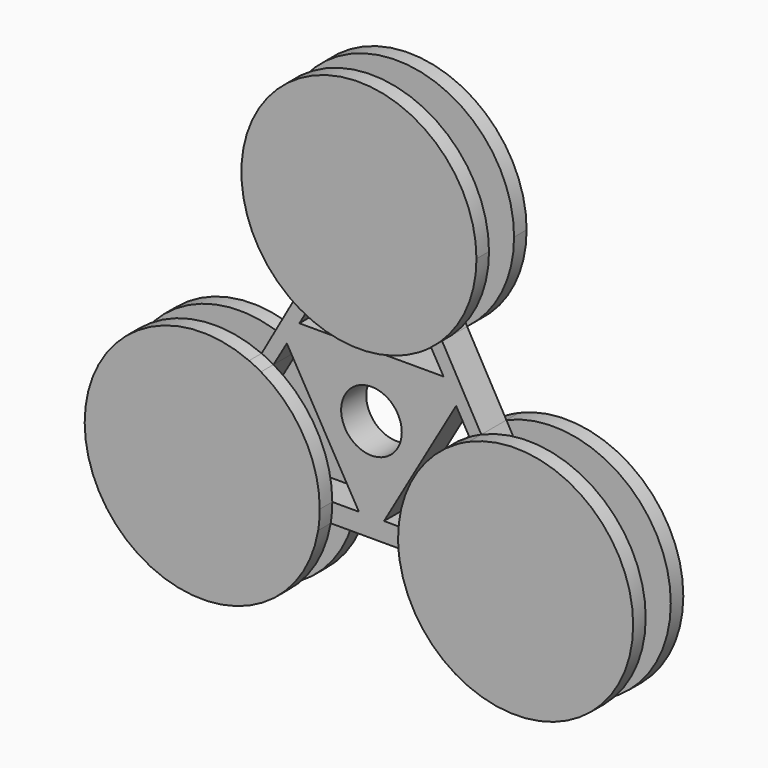
from build123d import *
from build123d import SkipClean  # not in build123d's __all__

# Parameters (mm, degrees)
F0_R     = 4.9113239183
F1_DEPTH = 5.08
F2_DEPTH = 2.54
F4_DEPTH = 2.54
F5_DEPTH = 5.08


# Not quite as in the source:
# - a feature names something its author has since deleted; it is built from what else it names


with BuildPart() as f1:
    # F0 (on Front) → F1 (new body)
    with BuildSketch(Plane.XZ):
        Polygon((11.684, -8.5716721153), (-11.684, -8.5716721153), (-12.7, -10.3314357358), (-13.716, -12.0911993563), (-2.032, -32.3284809919), (0, -32.3284809919), (2.032, -32.3284809919), (13.716, -12.0911993563), (12.7, -10.3314357358), align=None)
        with Locations((0, -18.7316721153)):
            Circle(F0_R, mode=Mode.SUBTRACT)
        with BuildLine():
            ThreePointArc((-11.4414768653, -3.5657760746), (-10.5023439874, -4.227888231), (-9.525, -4.8321744218))
            Line((-9.525, -4.8321744218), (0, 11.6656095203))
            Line((0, 11.6656095203), (0, 16.7456095203))
            Line((0, 16.7456095203), (-11.4414768653, -3.5657760746))
        make_face()
        with BuildLine():
            Line((9.525, -4.8321744218), (11.684, -8.5716721153))
            Line((11.684, -8.5716721153), (12.7, -10.3314357358))
            Line((12.7, -10.3314357358), (13.716, -12.0911993563))
            Line((13.716, -12.0911993563), (15.875, -15.8306970498))
            ThreePointArc((15.875, -15.8306970498), (16.8251832643, -15.3174546282), (17.8029235649, -14.8588808351))
            Line((17.8029235649, -14.8588808351), (11.4414768653, -3.5657760746))
            ThreePointArc((11.4414768653, -3.5657760746), (10.5023439874, -4.227888231), (9.525, -4.8321744218))
        make_face()
        with BuildLine():
            Line((0, 16.7456095203), (0, 11.6656095203))
            Line((0, 11.6656095203), (9.525, -4.8321744218))
            ThreePointArc((9.525, -4.8321744218), (10.5023439874, -4.227888231), (11.4414768653, -3.5657760746))
            Line((11.4414768653, -3.5657760746), (0, 16.7456095203))
        make_face()
        with BuildLine():
            Line((-25.4, -32.3284809919), (-15.875, -15.8306970498))
            ThreePointArc((-15.875, -15.8306970498), (-16.8251832643, -15.3174546282), (-17.8029235649, -14.8588808351))
            Line((-17.8029235649, -14.8588808351), (-29.4044214139, -35.4543423357))
            Line((-29.4044214139, -35.4543423357), (-25.4, -32.3284809919))
        make_face()
        with BuildLine():
            Line((0, -32.3284809919), (-2.032, -32.3284809919))
            Line((-2.032, -32.3284809919), (-6.35, -32.3284809919))
            ThreePointArc((-6.35, -32.3284809919), (-6.4146614456, -33.8967347902), (-6.6082068216, -35.4543423357))
            Line((-6.6082068216, -35.4543423357), (6.6082068216, -35.4543423357))
            ThreePointArc((6.6082068216, -35.4543423357), (6.4146614456, -33.8967347902), (6.35, -32.3284809919))
            Line((6.35, -32.3284809919), (2.032, -32.3284809919))
            Line((2.032, -32.3284809919), (0, -32.3284809919))
        make_face()
        with BuildLine():
            Line((-6.35, -32.3284809919), (-25.4, -32.3284809919))
            Line((-25.4, -32.3284809919), (-29.4044214139, -35.4543423357))
            Line((-29.4044214139, -35.4543423357), (-6.6082068216, -35.4543423357))
            ThreePointArc((-6.6082068216, -35.4543423357), (-6.4146614456, -33.8967347902), (-6.35, -32.3284809919))
        make_face()
        with BuildLine():
            Line((29.4044214139, -35.4543423357), (17.8029235649, -14.8588808351))
            ThreePointArc((17.8029235649, -14.8588808351), (16.8251832643, -15.3174546282), (15.875, -15.8306970498))
            Line((15.875, -15.8306970498), (25.4, -32.3284809919))
            Line((25.4, -32.3284809919), (29.4044214139, -35.4543423357))
        make_face()
        with BuildLine():
            ThreePointArc((6.35, -32.3284809919), (6.4146614456, -33.8967347902), (6.6082068216, -35.4543423357))
            Line((6.6082068216, -35.4543423357), (29.4044214139, -35.4543423357))
            Line((29.4044214139, -35.4543423357), (25.4, -32.3284809919))
            Line((25.4, -32.3284809919), (6.35, -32.3284809919))
        make_face()
    extrude(amount=F1_DEPTH)

    # F0 (on Front) → F2 (join)
    with BuildSketch(Plane.XZ):
        with BuildLine():
            ThreePointArc((19.05, 11.6656095203), (-8.5130008139, 28.7076550883), (-11.4414768653, -3.5657760746))
            Line((-11.4414768653, -3.5657760746), (0, 16.7456095203))
            Line((0, 16.7456095203), (11.4414768653, -3.5657760746))
            ThreePointArc((11.4414768653, -3.5657760746), (17.042045568, 3.1526087064), (19.05, 11.6656095203))
        make_face()
        with BuildLine():
            Line((0, 11.6656095203), (-9.525, -4.8321744218))
            ThreePointArc((-9.525, -4.8321744218), (0, -7.3843904797), (9.525, -4.8321744218))
            Line((9.525, -4.8321744218), (0, 11.6656095203))
        make_face()
        with BuildLine():
            Line((-29.4044214139, -35.4543423357), (-17.8029235649, -14.8588808351))
            ThreePointArc((-17.8029235649, -14.8588808351), (-42.1372748222, -41.4260703169), (-6.6082068216, -35.4543423357))
            Line((-6.6082068216, -35.4543423357), (-29.4044214139, -35.4543423357))
        make_face()
        with BuildLine():
            ThreePointArc((-6.35, -32.3284809919), (-8.9022160579, -22.8034809919), (-15.875, -15.8306970498))
            Line((-15.875, -15.8306970498), (-25.4, -32.3284809919))
            Line((-25.4, -32.3284809919), (-6.35, -32.3284809919))
        make_face()
        with BuildLine():
            ThreePointArc((44.45, -32.3284809919), (35.8445726076, -16.3969586841), (17.8029235649, -14.8588808351))
            Line((17.8029235649, -14.8588808351), (29.4044214139, -35.4543423357))
            Line((29.4044214139, -35.4543423357), (6.6082068216, -35.4543423357))
            ThreePointArc((6.6082068216, -35.4543423357), (26.9682537983, -51.3138195463), (44.45, -32.3284809919))
        make_face()
        with BuildLine():
            Line((25.4, -32.3284809919), (15.875, -15.8306970498))
            ThreePointArc((15.875, -15.8306970498), (8.9022160579, -22.8034809919), (6.35, -32.3284809919))
            Line((6.35, -32.3284809919), (25.4, -32.3284809919))
        make_face()
        with BuildLine():
            Line((-6.35, -32.3284809919), (-25.4, -32.3284809919))
            Line((-25.4, -32.3284809919), (-29.4044214139, -35.4543423357))
            Line((-29.4044214139, -35.4543423357), (-6.6082068216, -35.4543423357))
            ThreePointArc((-6.6082068216, -35.4543423357), (-6.4146614456, -33.8967347902), (-6.35, -32.3284809919))
        make_face()
        with BuildLine():
            Line((-25.4, -32.3284809919), (-15.875, -15.8306970498))
            ThreePointArc((-15.875, -15.8306970498), (-16.8251832643, -15.3174546282), (-17.8029235649, -14.8588808351))
            Line((-17.8029235649, -14.8588808351), (-29.4044214139, -35.4543423357))
            Line((-29.4044214139, -35.4543423357), (-25.4, -32.3284809919))
        make_face()
        with BuildLine():
            ThreePointArc((6.35, -32.3284809919), (6.4146614456, -33.8967347902), (6.6082068216, -35.4543423357))
            Line((6.6082068216, -35.4543423357), (29.4044214139, -35.4543423357))
            Line((29.4044214139, -35.4543423357), (25.4, -32.3284809919))
            Line((25.4, -32.3284809919), (6.35, -32.3284809919))
        make_face()
        with BuildLine():
            Line((29.4044214139, -35.4543423357), (17.8029235649, -14.8588808351))
            ThreePointArc((17.8029235649, -14.8588808351), (16.8251832643, -15.3174546282), (15.875, -15.8306970498))
            Line((15.875, -15.8306970498), (25.4, -32.3284809919))
            Line((25.4, -32.3284809919), (29.4044214139, -35.4543423357))
        make_face()
        with BuildLine():
            Line((0, 16.7456095203), (0, 11.6656095203))
            Line((0, 11.6656095203), (9.525, -4.8321744218))
            ThreePointArc((9.525, -4.8321744218), (10.5023439874, -4.227888231), (11.4414768653, -3.5657760746))
            Line((11.4414768653, -3.5657760746), (0, 16.7456095203))
        make_face()
        with BuildLine():
            ThreePointArc((-11.4414768653, -3.5657760746), (-10.5023439874, -4.227888231), (-9.525, -4.8321744218))
            Line((-9.525, -4.8321744218), (0, 11.6656095203))
            Line((0, 11.6656095203), (0, 16.7456095203))
            Line((0, 16.7456095203), (-11.4414768653, -3.5657760746))
        make_face()
    extrude(amount=-F2_DEPTH)

    # F3 (on face) → F4 (join)
    with BuildSketch(Plane.XZ.offset(5.08)):
        with BuildLine():
            ThreePointArc((11.4414768653, -3.5657760746), (17.042045568, 3.1526087064), (19.05, 11.6656095203))
            ThreePointArc((19.05, 11.6656095203), (-8.5130008139, 28.7076550883), (-11.4414768653, -3.5657760746))
            Line((-11.4414768653, -3.5657760746), (0, 16.7456095203))
            Line((0, 16.7456095203), (11.4414768653, -3.5657760746))
        make_face()
        with BuildLine():
            Line((0, 16.7456095203), (-11.4414768653, -3.5657760746))
            ThreePointArc((-11.4414768653, -3.5657760746), (-10.5023439874, -4.227888231), (-9.525, -4.8321744218))
            Line((-9.525, -4.8321744218), (0, 11.6656095203))
            Line((0, 11.6656095203), (9.525, -4.8321744218))
            ThreePointArc((9.525, -4.8321744218), (10.5023439874, -4.227888231), (11.4414768653, -3.5657760746))
            Line((11.4414768653, -3.5657760746), (0, 16.7456095203))
        make_face()
        with BuildLine():
            Line((0, 11.6656095203), (-9.525, -4.8321744218))
            ThreePointArc((-9.525, -4.8321744218), (0, -7.3843904797), (9.525, -4.8321744218))
            Line((9.525, -4.8321744218), (0, 11.6656095203))
        make_face()
        with BuildLine():
            Line((29.4044214139, -35.4543423357), (17.8029235649, -14.8588808351))
            ThreePointArc((17.8029235649, -14.8588808351), (16.8251832643, -15.3174546282), (15.875, -15.8306970498))
            Line((15.875, -15.8306970498), (25.4, -32.3284809919))
            Line((25.4, -32.3284809919), (6.35, -32.3284809919))
            ThreePointArc((6.35, -32.3284809919), (6.4146614456, -33.8967347902), (6.6082068216, -35.4543423357))
            Line((6.6082068216, -35.4543423357), (29.4044214139, -35.4543423357))
        make_face()
        with BuildLine():
            ThreePointArc((44.45, -32.3284809919), (35.8445726076, -16.3969586841), (17.8029235649, -14.8588808351))
            Line((17.8029235649, -14.8588808351), (29.4044214139, -35.4543423357))
            Line((29.4044214139, -35.4543423357), (6.6082068216, -35.4543423357))
            ThreePointArc((6.6082068216, -35.4543423357), (26.9682537983, -51.3138195463), (44.45, -32.3284809919))
        make_face()
        with BuildLine():
            Line((25.4, -32.3284809919), (15.875, -15.8306970498))
            ThreePointArc((15.875, -15.8306970498), (8.9022160579, -22.8034809919), (6.35, -32.3284809919))
            Line((6.35, -32.3284809919), (25.4, -32.3284809919))
        make_face()
        with BuildLine():
            Line((-29.4044214139, -35.4543423357), (-6.6082068216, -35.4543423357))
            ThreePointArc((-6.6082068216, -35.4543423357), (-6.4146614456, -33.8967347902), (-6.35, -32.3284809919))
            Line((-6.35, -32.3284809919), (-25.4, -32.3284809919))
            Line((-25.4, -32.3284809919), (-15.875, -15.8306970498))
            ThreePointArc((-15.875, -15.8306970498), (-16.8251832643, -15.3174546282), (-17.8029235649, -14.8588808351))
            Line((-17.8029235649, -14.8588808351), (-29.4044214139, -35.4543423357))
        make_face()
        with BuildLine():
            ThreePointArc((-17.8029235649, -14.8588808351), (-42.1372748222, -41.4260703169), (-6.6082068216, -35.4543423357))
            Line((-6.6082068216, -35.4543423357), (-29.4044214139, -35.4543423357))
            Line((-29.4044214139, -35.4543423357), (-17.8029235649, -14.8588808351))
        make_face()
        with BuildLine():
            Line((-25.4, -32.3284809919), (-6.35, -32.3284809919))
            ThreePointArc((-6.35, -32.3284809919), (-8.9022160579, -22.8034809919), (-15.875, -15.8306970498))
            Line((-15.875, -15.8306970498), (-25.4, -32.3284809919))
        make_face()
    with SkipClean():  # cleaning this boolean's faces spoils the solid; the shape is the same uncleaned
        extrude(amount=F4_DEPTH)

    # F0 (on Front) → F5 (join)
    with BuildSketch(Plane.XZ):
        Polygon((11.684, -8.5716721153), (-11.684, -8.5716721153), (-12.7, -10.3314357358), (-13.716, -12.0911993563), (-2.032, -32.3284809919), (0, -32.3284809919), (2.032, -32.3284809919), (13.716, -12.0911993563), (12.7, -10.3314357358), align=None)
        with Locations((0, -18.7316721153)):
            Circle(F0_R, mode=Mode.SUBTRACT)
        with BuildLine():
            Line((-12.7, -10.3314357358), (-11.684, -8.5716721153))
            Line((-11.684, -8.5716721153), (-9.525, -4.8321744218))
            ThreePointArc((-9.525, -4.8321744218), (-10.5023439874, -4.227888231), (-11.4414768653, -3.5657760746))
            Line((-11.4414768653, -3.5657760746), (-17.8029235649, -14.8588808351))
            ThreePointArc((-17.8029235649, -14.8588808351), (-16.8251832643, -15.3174546282), (-15.875, -15.8306970498))
            Line((-15.875, -15.8306970498), (-13.716, -12.0911993563))
            Line((-13.716, -12.0911993563), (-12.7, -10.3314357358))
        make_face()
    extrude(amount=F5_DEPTH)


solid = f1.part
